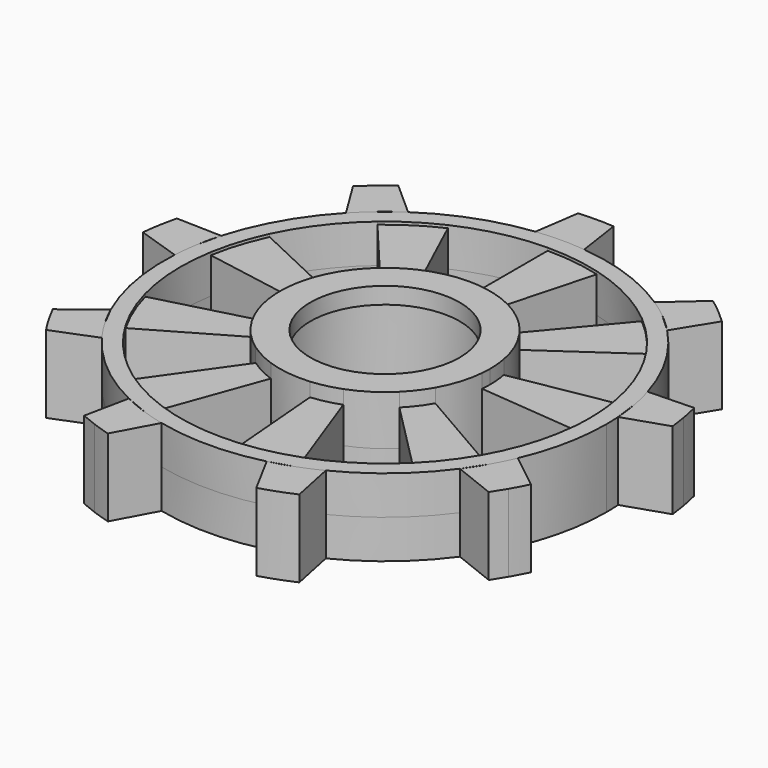
from build123d import *

# Parameters (mm, degrees)
F0_R     = 8
F1_DEPTH = 4.5
F2_DEPTH = 3.25
F3_DEPTH = 3.5
F4_DEPTH = 3.5
F5_R     = 8
F5_R_2   = 6.75
F6_DEPTH = 1.5


# Not quite as in the source:
# - a feature names something its author has since deleted; it is built from what else it names


with BuildPart() as f1:
    # F0 (on Top) → F1 (new body, symmetric)
    with BuildSketch(Plane.XY):
        with BuildLine():
            ThreePointArc((9.4605594205, -0.8647632344), (9.4901347328, -0.4328310903), (9.5, 0))
            ThreePointArc((9.5, 0), (9.4593543355, 0.8778471143), (9.3377651461, 1.7481825066))
            ThreePointArc((9.3377651461, 1.7481825066), (8.7647124781, 3.6646712235), (7.8030680653, 5.4186833058))
            ThreePointArc((7.8030680653, 5.4186833058), (6.9827442619, 6.4413727243), (6.0294330466, 7.3413852328))
            ThreePointArc((6.0294330466, 7.3413852328), (4.3585540334, 8.44114961), (2.4944344409, 9.1666677053))
            ThreePointArc((2.4944344409, 9.1666677053), (1.208657863, 9.4227992746), (-0.1001377851, 9.4994722182))
            ThreePointArc((-0.1001377851, 9.4994722182), (-2.0870202835, 9.2679202811), (-3.981372781, 8.6254664094))
            ThreePointArc((-3.981372781, 8.6254664094), (-5.1309729827, 7.9951933217), (-6.1828530342, 7.2126505778))
            ThreePointArc((-6.1828530342, 7.2126505778), (-7.5560546151, 5.7581280512), (-8.5942514305, 4.048313519))
            ThreePointArc((-8.5942514305, 4.048313519), (-9.0697645454, 2.8265475568), (-9.3725426339, 1.5509495723))
            ThreePointArc((-9.3725426339, 1.5509495723), (-9.4895270161, -0.4459562883), (-9.1857843213, -2.4230902588))
            ThreePointArc((-9.1857843213, -2.4230902588), (-8.7647124781, -3.6646712235), (-8.1767153709, -4.8364579749))
            ThreePointArc((-8.1767153709, -4.8364579749), (-6.9827442619, -6.4413727243), (-5.4791866395, -7.7607031749))
            ThreePointArc((-5.4791866395, -7.7607031749), (-4.3585540334, -8.44114961), (-3.1549121119, -8.9608330844))
            ThreePointArc((-3.1549121119, -8.9608330844), (-1.208657863, -9.4227992746), (0.7911833653, -9.4669968249))
            ThreePointArc((0.7911833653, -9.4669968249), (2.0870202835, -9.2679202811), (3.3431095873, -8.8923348052))
            ThreePointArc((3.3431095873, -8.8923348052), (5.1309729827, -7.9951933217), (6.6913498805, -6.7435774465))
            ThreePointArc((6.6913498805, -6.7435774465), (7.5560546151, -5.7581280512), (8.276853156, -4.6630142433))
            ThreePointArc((8.276853156, -4.6630142433), (9.0697645454, -2.8265475568), (9.4605594205, -0.8647632344))
        make_face()
        Circle(F0_R, mode=Mode.SUBTRACT)
    extrude(amount=F1_DEPTH, both=True)

    # F5 (on face) → F6 (join)
    with BuildSketch(Plane.XY.offset(4.5)):
        Circle(F5_R)
        Circle(F5_R_2, mode=Mode.SUBTRACT)
    extrude(amount=-F6_DEPTH)


with BuildPart() as f2:
    # F0 (on Top) → F2 (new body, symmetric)
    with BuildSketch(Plane.XY):
        with BuildLine():
            ThreePointArc((-6.1828530342, 7.2126505778), (-5.1309729827, 7.9951933217), (-3.981372781, 8.6254664094))
            Line((-3.981372781, 8.6254664094), (-7.7531996261, 16.7969609024))
            ThreePointArc((-7.7531996261, 16.7969609024), (-9.9519404819, 15.5951556788), (-11.9681065663, 14.1072472587))
            Line((-11.9681065663, 14.1072472587), (-6.1828530342, 7.2126505778))
        make_face()
    extrude(amount=F2_DEPTH, both=True)


with BuildPart() as f2b:
    # F0 (on Top) → F2, piece 2 (new body, symmetric)
    with BuildSketch(Plane.XY):
        with BuildLine():
            ThreePointArc((-0.1001377851, 9.4994722182), (1.208657863, 9.4227992746), (2.4944344409, 9.1666677053))
            Line((2.4944344409, 9.1666677053), (4.8575828585, 17.8508792157))
            ThreePointArc((4.8575828585, 17.8508792157), (2.400744137, 18.3435663814), (-0.1001377851, 18.4997289824))
            Line((-0.1001377851, 18.4997289824), (-0.1001377851, 9.4994722182))
        make_face()
    extrude(amount=F2_DEPTH, both=True)


with BuildPart() as f2c:
    # F0 (on Top) → F2, piece 3 (new body, symmetric)
    with BuildSketch(Plane.XY):
        with BuildLine():
            ThreePointArc((6.0294330466, 7.3413852328), (6.9827442619, 6.4413727243), (7.8030680653, 5.4186833058))
            Line((7.8030680653, 5.4186833058), (15.1954483376, 10.5521727535))
            ThreePointArc((15.1954483376, 10.5521727535), (13.630093893, 12.5088185081), (11.8146865786, 14.2359819137))
            Line((11.8146865786, 14.2359819137), (6.0294330466, 7.3413852328))
        make_face()
    extrude(amount=F2_DEPTH, both=True)


with BuildPart() as f2d:
    # F0 (on Top) → F2, piece 4 (new body, symmetric)
    with BuildSketch(Plane.XY):
        with BuildLine():
            ThreePointArc((9.3377651461, 1.7481825066), (9.4593543355, 0.8778471143), (9.5, 0))
            ThreePointArc((9.5, 0), (9.4901347328, -0.4328310903), (9.4605594205, -0.8647632344))
            Line((9.4605594205, -0.8647632344), (18.4231946609, -1.6840126144))
            ThreePointArc((18.4231946609, -1.6840126144), (18.4807886902, -0.8428815969), (18.5, 0))
            ThreePointArc((18.5, 0), (18.4251706105, 1.6622538836), (18.2012877866, 3.3110606923))
            Line((18.2012877866, 3.3110606923), (9.3377651461, 1.7481825066))
        make_face()
    extrude(amount=F2_DEPTH, both=True)


with BuildPart() as f2e:
    # F0 (on Top) → F2, piece 5 (new body, symmetric)
    with BuildSketch(Plane.XY):
        with BuildLine():
            Line((16.0713041545, -9.1631426254), (8.276853156, -4.6630142433))
            ThreePointArc((8.276853156, -4.6630142433), (7.5560546151, -5.7581280512), (6.6913498805, -6.7435774465))
            Line((6.6913498805, -6.7435774465), (13.0305234514, -13.1322297643))
            ThreePointArc((13.0305234514, -13.1322297643), (14.6856224138, -11.2508886014), (16.0713041545, -9.1631426254))
        make_face()
    extrude(amount=F2_DEPTH, both=True)


with BuildPart() as f2f:
    # F0 (on Top) → F2, piece 6 (new body, symmetric)
    with BuildSketch(Plane.XY):
        with BuildLine():
            Line((6.4213786958, -17.3498096717), (3.3431095873, -8.8923348052))
            ThreePointArc((3.3431095873, -8.8923348052), (2.0870202835, -9.2679202811), (0.7911833653, -9.4669968249))
            Line((0.7911833653, -9.4669968249), (1.5407255008, -18.435730659))
            ThreePointArc((1.5407255008, -18.435730659), (4.0179076529, -18.0584168213), (6.4213786958, -17.3498096717))
        make_face()
    extrude(amount=F2_DEPTH, both=True)


with BuildPart() as f2g:
    # F0 (on Top) → F2, piece 7 (new body, symmetric)
    with BuildSketch(Plane.XY):
        with BuildLine():
            Line((-6.2331812203, -17.418307951), (-3.1549121119, -8.9608330844))
            ThreePointArc((-3.1549121119, -8.9608330844), (-4.3585540334, -8.44114961), (-5.4791866395, -7.7607031749))
            Line((-5.4791866395, -7.7607031749), (-10.6699950348, -15.112948288))
            ThreePointArc((-10.6699950348, -15.112948288), (-8.5298307528, -16.4162111136), (-6.2331812203, -17.418307951))
        make_face()
    extrude(amount=F2_DEPTH, both=True)


with BuildPart() as f2h:
    # F0 (on Top) → F2, piece 8 (new body, symmetric)
    with BuildSketch(Plane.XY):
        with BuildLine():
            Line((-15.9711663694, -9.336586357), (-8.1767153709, -4.8364579749))
            ThreePointArc((-8.1767153709, -4.8364579749), (-8.7647124781, -3.6646712235), (-9.1857843213, -2.4230902588))
            Line((-9.1857843213, -2.4230902588), (-17.8881063099, -4.7186494514))
            ThreePointArc((-17.8881063099, -4.7186494514), (-17.0863665508, -7.09267778), (-15.9711663694, -9.336586357))
        make_face()
    extrude(amount=F2_DEPTH, both=True)


with BuildPart() as f2i:
    # F0 (on Top) → F2, piece 9 (new body, symmetric)
    with BuildSketch(Plane.XY):
        with BuildLine():
            ThreePointArc((-9.3725426339, 1.5509495723), (-9.0697645454, 2.8265475568), (-8.5942514305, 4.048313519))
            Line((-8.5942514305, 4.048313519), (-16.7361738384, 7.8835579055))
            ThreePointArc((-16.7361738384, 7.8835579055), (-17.6480015458, 5.5495983132), (-18.2360652744, 3.113827758))
            Line((-18.2360652744, 3.113827758), (-9.3725426339, 1.5509495723))
        make_face()
    extrude(amount=F2_DEPTH, both=True)


with BuildPart() as f3:
    # F0 (on Top) → F3 (new body, symmetric)
    with BuildSketch(Plane.XY):
        with BuildLine():
            ThreePointArc((-2.295447708, 19.8678363145), (-0.0997720274, 19.999751137), (2.097110494, 19.889749309))
            Line((2.097110494, 19.889749309), (1.4992673992, 23.953125))
            ThreePointArc((1.4992673992, 23.953125), (-0.0998875357, 23.9997921341), (-1.6985986171, 23.9398154282))
            Line((-1.6985986171, 23.9398154282), (-2.295447708, 19.8678363145))
        make_face()
    extrude(amount=F3_DEPTH, both=True)


with BuildPart() as f3b:
    # F0 (on Top) → F3, piece 2 (new body, symmetric)
    with BuildSketch(Plane.XY):
        with BuildLine():
            ThreePointArc((12.7788810589, 15.3850641495), (13.6057168905, 14.6589381572), (14.3913642561, 13.8884352915))
            Line((14.3913642561, 13.8884352915), (16.5452774232, 17.3854477938))
            Line((16.5452774232, 17.3854477938), (15.4269026325, 18.3850666349))
            ThreePointArc((15.4269026325, 18.3850666349), (14.7662188484, 18.9197986491), (14.0870147037, 19.430800723))
            Line((14.0870147037, 19.430800723), (11.0123840531, 16.6951309509))
            ThreePointArc((11.0123840531, 16.6951309509), (11.9136536236, 16.0643971981), (12.7788810589, 15.3850641495))
        make_face()
    extrude(amount=F3_DEPTH, both=True)


with BuildPart() as f3c:
    # F0 (on Top) → F3, piece 3 (new body, symmetric)
    with BuildSketch(Plane.XY):
        with BuildLine():
            ThreePointArc((19.6785194339, 3.5715364885), (19.8451676372, 2.4838118792), (19.9517387406, 1.3885680484))
            Line((19.9517387406, 1.3885680484), (23.8495682606, 2.6829263471))
            Line((23.8495682606, 2.6829263471), (23.6353860723, 4.167556264))
            ThreePointArc((23.6353860723, 4.167556264), (23.4729920441, 5.0018641024), (23.281157285, 5.8298984102))
            Line((23.281157285, 5.8298984102), (19.1673989267, 5.7105882696))
            ThreePointArc((19.1673989267, 5.7105882696), (19.4523836316, 4.6480932703), (19.6785194339, 3.5715364885))
        make_face()
    extrude(amount=F3_DEPTH, both=True)


with BuildPart() as f3d:
    # F0 (on Top) → F3, piece 4 (new body, symmetric)
    with BuildSketch(Plane.XY):
        with BuildLine():
            Line((21.5817876313, -10.4988781609), (18.3537748206, -7.9460021291))
            ThreePointArc((18.3537748206, -7.9460021291), (17.8891271492, -8.9431051564), (17.3703598635, -9.9131527887))
            ThreePointArc((17.3703598635, -9.9131527887), (16.798843892, -10.8535175815), (16.1764729295, -11.7610256169))
            Line((16.1764729295, -11.7610256169), (19.9943810504, -13.2749661548))
            Line((19.9943810504, -13.2749661548), (20.7846096908, -12))
            ThreePointArc((20.7846096908, -12), (21.1964913891, -11.2564982473), (21.5817876313, -10.4988781609))
        make_face()
    extrude(amount=F3_DEPTH, both=True)


with BuildPart() as f3e:
    # F0 (on Top) → F3, piece 5 (new body, symmetric)
    with BuildSketch(Plane.XY):
        with BuildLine():
            Line((9.7840596901, -21.9151129584), (8.9522154964, -17.8845698216))
            ThreePointArc((8.9522154964, -17.8845698216), (7.9553492582, -18.3497252889), (6.9344158629, -18.7593677036))
            ThreePointArc((6.9344158629, -18.7593677036), (5.8921543914, -19.1123655424), (4.8320556532, -19.4075046867))
            Line((4.8320556532, -19.4075046867), (6.783600734, -23.021354458))
            ThreePointArc((6.783600734, -23.021354458), (8.3022759257, -22.5182640195), (9.7840596901, -21.9151129584))
        make_face()
    extrude(amount=F3_DEPTH, both=True)


with BuildPart() as f3f:
    # F0 (on Top) → F3, piece 6 (new body, symmetric)
    with BuildSketch(Plane.XY):
        with BuildLine():
            Line((-6.5917385178, -23.0770228434), (-4.6381849513, -19.4547485298))
            ThreePointArc((-4.6381849513, -19.4547485298), (-5.7008249645, -19.1703050243), (-6.7462183874, -18.8278659829))
            ThreePointArc((-6.7462183874, -18.8278659829), (-7.771539633, -18.4283252558), (-8.7733341656, -17.9729966233))
            Line((-8.7733341656, -17.9729966233), (-9.6013017572, -21.9957951565))
            Line((-9.6013017572, -21.9957951565), (-8.2084834398, -22.5526228989))
            ThreePointArc((-8.2084834398, -22.5526228989), (-7.4047546431, -22.8291394642), (-6.5917385178, -23.0770228434))
        make_face()
    extrude(amount=F3_DEPTH, both=True)


with BuildPart() as f3g:
    # F0 (on Top) → F3, piece 7 (new body, symmetric)
    with BuildSketch(Plane.XY):
        with BuildLine():
            Line((-19.8831890142, -13.4409372674), (-16.0583271126, -11.9218341854))
            ThreePointArc((-16.0583271126, -11.9218341854), (-16.6895198288, -11.0208859845), (-17.2702220784, -10.0865965203))
            ThreePointArc((-17.2702220784, -10.0865965203), (-17.798843892, -9.1214667739), (-18.2735834235, -8.1287236922))
            Line((-18.2735834235, -8.1287236922), (-21.4936484496, -10.6781588452))
            Line((-21.4936484496, -10.6781588452), (-20.7846096908, -12))
            ThreePointArc((-20.7846096908, -12), (-20.3466591344, -12.7284508904), (-19.8831890142, -13.4409372674))
        make_face()
    extrude(amount=F3_DEPTH, both=True)


with BuildPart() as f3h:
    # F0 (on Top) → F3, piece 8 (new body, symmetric)
    with BuildSketch(Plane.XY):
        with BuildLine():
            ThreePointArc((-19.7132969217, 3.3743035542), (-19.4978712819, 4.4534273853), (-19.2234199094, 5.5190693952))
            Line((-19.2234199094, 5.5190693952), (-23.3288781572, 5.6359066643))
            Line((-23.3288781572, 5.6359066643), (-23.6353860723, 4.167556264))
            ThreePointArc((-23.6353860723, 4.167556264), (-23.7681356888, 3.328021316), (-23.8710743939, 2.4843122354))
            Line((-23.8710743939, 2.4843122354), (-19.9645995495, 1.1894388707))
            ThreePointArc((-19.9645995495, 1.1894388707), (-19.8690028818, 2.2853280909), (-19.7132969217, 3.3743035542))
        make_face()
    extrude(amount=F3_DEPTH, both=True)


with BuildPart() as f3i:
    # F0 (on Top) → F3, piece 9 (new body, symmetric)
    with BuildSketch(Plane.XY):
        with BuildLine():
            ThreePointArc((-12.9323010465, 15.2563294944), (-12.0736280042, 15.9445133766), (-11.1784045751, 16.5844285749))
            Line((-11.1784045751, 16.5844285749), (-14.2482665033, 19.3128688094))
            Line((-14.2482665033, 19.3128688094), (-15.4269026325, 18.3850666349))
            ThreePointArc((-15.4269026325, 18.3850666349), (-16.068237401, 17.8272753618), (-16.6894187672, 17.2471244332))
            Line((-16.6894187672, 17.2471244332), (-14.5292139754, 13.7441602602))
            ThreePointArc((-14.5292139754, 13.7441602602), (-13.751558667, 14.522211754), (-12.9323010465, 15.2563294944))
        make_face()
    extrude(amount=F3_DEPTH, both=True)


with BuildPart() as f4:
    # F0 (on Top) → F4 (new body, symmetric)
    with BuildSketch(Plane.XY):
        with BuildLine():
            ThreePointArc((18.3537748206, -7.9460021291), (19.5841197966, -4.0573700588), (20, 0))
            ThreePointArc((20, 0), (19.9879310437, 0.6947032413), (19.9517387406, 1.3885680484))
            Line((19.9517387406, 1.3885680484), (19.6785194339, 3.5715364885))
            ThreePointArc((19.6785194339, 3.5715364885), (19.4523836316, 4.6480932703), (19.1673989267, 5.7105882696))
            ThreePointArc((19.1673989267, 5.7105882696), (17.2704065403, 10.0862806788), (14.3913642561, 13.8884352915))
            Line((14.3913642561, 13.8884352915), (12.7788810589, 15.3850641495))
            ThreePointArc((12.7788810589, 15.3850641495), (11.9136536236, 16.0643971981), (11.0123840531, 16.6951309509))
            ThreePointArc((11.0123840531, 16.6951309509), (6.7465627125, 18.8277426041), (2.097110494, 19.889749309))
            ThreePointArc((2.097110494, 19.889749309), (-0.0997720274, 19.999751137), (-2.295447708, 19.8678363145))
            ThreePointArc((-2.295447708, 19.8678363145), (-6.9340727882, 18.7594945179), (-11.1784045751, 16.5844285749))
            Line((-11.1784045751, 16.5844285749), (-12.9323010465, 15.2563294944))
            ThreePointArc((-12.9323010465, 15.2563294944), (-13.751558667, 14.522211754), (-14.5292139754, 13.7441602602))
            ThreePointArc((-14.5292139754, 13.7441602602), (-17.3701785677, 9.9134704582), (-19.2234199094, 5.5190693952))
            Line((-19.2234199094, 5.5190693952), (-19.7132969217, 3.3743035542))
            ThreePointArc((-19.7132969217, 3.3743035542), (-19.8690028818, 2.2853280909), (-19.9645995495, 1.1894388707))
            ThreePointArc((-19.9645995495, 1.1894388707), (-19.6785847473, -3.5711766048), (-18.2735834235, -8.1287236922))
            Line((-18.2735834235, -8.1287236922), (-17.2702220784, -10.0865965203))
            ThreePointArc((-17.2702220784, -10.0865965203), (-16.6895198288, -11.0208859845), (-16.0583271126, -11.9218341854))
            ThreePointArc((-16.0583271126, -11.9218341854), (-12.7791624205, -15.3848304453), (-8.7733341656, -17.9729966233))
            Line((-8.7733341656, -17.9729966233), (-6.7462183874, -18.8278659829))
            ThreePointArc((-6.7462183874, -18.8278659829), (-5.7008249645, -19.1703050243), (-4.6381849513, -19.4547485298))
            ThreePointArc((-4.6381849513, -19.4547485298), (0.0997720274, -19.999751137), (4.8320556532, -19.4075046867))
            Line((4.8320556532, -19.4075046867), (6.9344158629, -18.7593677036))
            ThreePointArc((6.9344158629, -18.7593677036), (7.9553492582, -18.3497252889), (8.9522154964, -17.8845698216))
            ThreePointArc((8.9522154964, -17.8845698216), (12.9320220348, -15.2565659993), (16.1764729295, -11.7610256169))
            Line((16.1764729295, -11.7610256169), (17.3703598635, -9.9131527887))
            ThreePointArc((17.3703598635, -9.9131527887), (17.8891271492, -8.9431051564), (18.3537748206, -7.9460021291))
        make_face()
        with BuildLine():
            ThreePointArc((15.1954483376, 10.5521727535), (17.0863665508, 7.09267778), (18.2012877866, 3.3110606923))
            ThreePointArc((18.2012877866, 3.3110606923), (18.4251706105, 1.6622538836), (18.5, 0))
            ThreePointArc((18.5, 0), (18.4807886902, -0.8428815969), (18.4231946609, -1.6840126144))
            ThreePointArc((18.4231946609, -1.6840126144), (17.6480015458, -5.5495983132), (16.0713041545, -9.1631426254))
            ThreePointArc((16.0713041545, -9.1631426254), (14.6856224138, -11.2508886014), (13.0305234514, -13.1322297643))
            ThreePointArc((13.0305234514, -13.1322297643), (9.9519404819, -15.5951556788), (6.4213786958, -17.3498096717))
            ThreePointArc((6.4213786958, -17.3498096717), (4.0179076529, -18.0584168213), (1.5407255008, -18.435730659))
            ThreePointArc((1.5407255008, -18.435730659), (-2.400744137, -18.3435663814), (-6.2331812203, -17.418307951))
            ThreePointArc((-6.2331812203, -17.418307951), (-8.5298307528, -16.4162111136), (-10.6699950348, -15.112948288))
            ThreePointArc((-10.6699950348, -15.112948288), (-13.630093893, -12.5088185081), (-15.9711663694, -9.336586357))
            ThreePointArc((-15.9711663694, -9.336586357), (-17.0863665508, -7.09267778), (-17.8881063099, -4.7186494514))
            ThreePointArc((-17.8881063099, -4.7186494514), (-18.4817712347, -0.8210554349), (-18.2360652744, 3.113827758))
            ThreePointArc((-18.2360652744, 3.113827758), (-17.6480015458, 5.5495983132), (-16.7361738384, 7.8835579055))
            ThreePointArc((-16.7361738384, 7.8835579055), (-14.6856224138, 11.2508886014), (-11.9681065663, 14.1072472587))
            ThreePointArc((-11.9681065663, 14.1072472587), (-9.9519404819, 15.5951556788), (-7.7531996261, 16.7969609024))
            ThreePointArc((-7.7531996261, 16.7969609024), (-4.0179076529, 18.0584168213), (-0.1001377851, 18.4997289824))
            ThreePointArc((-0.1001377851, 18.4997289824), (2.400744137, 18.3435663814), (4.8575828585, 17.8508792157))
            ThreePointArc((4.8575828585, 17.8508792157), (8.5298307528, 16.4162111136), (11.8146865786, 14.2359819137))
            ThreePointArc((11.8146865786, 14.2359819137), (13.630093893, 12.5088185081), (15.1954483376, 10.5521727535))
        make_face(mode=Mode.SUBTRACT)
    extrude(amount=F4_DEPTH, both=True)


solid = Compound([f1.part, f2.part, f2b.part, f2c.part, f2d.part, f2e.part, f2f.part, f2g.part, f2h.part, f2i.part, f3.part, f3b.part, f3c.part, f3d.part, f3e.part, f3f.part, f3g.part, f3h.part, f3i.part, f4.part])
